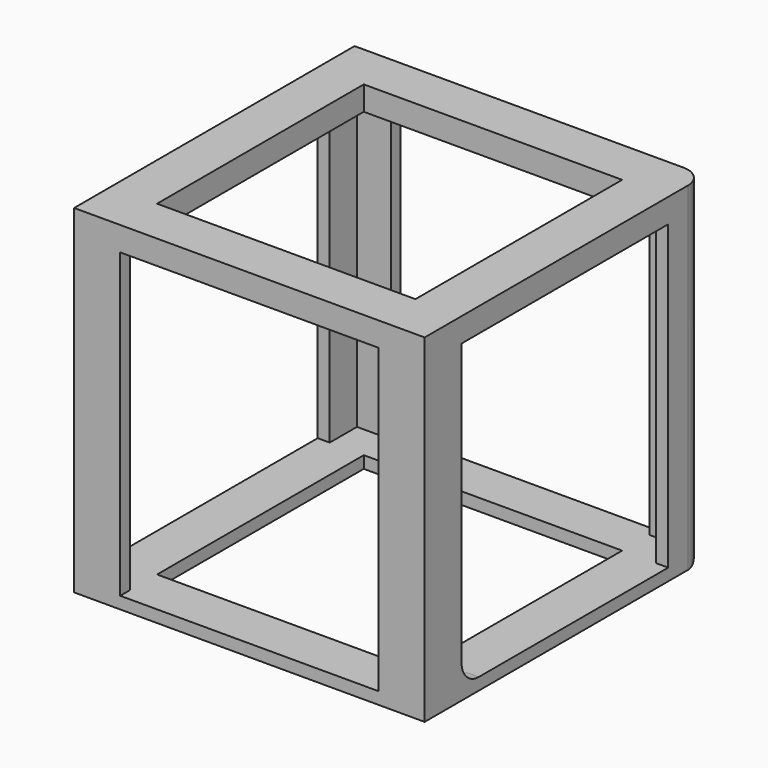
from build123d import *

# Parameters (mm, degrees)
F0_W        = 60
F0_H        = 2.8
F0_W_2      = 2.8
F0_H_2      = 60
F0_W_3      = 7.9
F0_H_3      = 7.9
F1_DEPTH    = 75.8
F2_DEPTH    = 70.2
F3_DEPTH    = 75.8
F4_DEPTH    = 2.8
F5_T1_DEPTH = 2.8
F5_T3_DEPTH = 106.4
F5_T5_DEPTH = 103.6


# Not quite as in the source:
# - a fillet or chamfer that OpenCascade refuses, or shapes differently, is made with other operations: its cross-section is extruded or revolved along the edge and cut away or added


with BuildPart() as f1:
    # F0 (on Top) → F1 (new body)
    with BuildSketch(Plane.XY):
        with Locations((0, 39.3)):
            Rectangle(F0_W, F0_H)
        Polygon((-40.7, 30), (-37.9, 30), (-37.9, 37.9), (-30, 37.9), (-30, 40.7), (-40.7, 40.7), align=None)
        Polygon((37.9, 37.9), (37.9, 30), (40.7, 30), (40.7, 40.7), (30, 40.7), (30, 37.9), align=None)
        with Locations((39.3, 0)):
            Rectangle(F0_W_2, F0_H_2)
        Polygon((37.9, -30), (37.9, -37.9), (30, -37.9), (30, -40.7), (40.7, -40.7), (40.7, -30), align=None)
        with Locations((0, -39.3)):
            Rectangle(F0_W, F0_H)
        Polygon((-30, -40.7), (-30, -37.9), (-37.9, -37.9), (-37.9, -30), (-40.7, -30), (-40.7, -40.7), align=None)
        with Locations((-39.3, 0)):
            Rectangle(F0_W_2, F0_H_2)
        with Locations((33.95, -33.95)):
            Rectangle(F0_W_3, F0_H_3)
        with Locations((33.95, 33.95)):
            Rectangle(F0_W_3, F0_H_3)
        with Locations((-33.95, 33.95)):
            Rectangle(F0_W_3, F0_H_3)
        with Locations((-33.95, 0)):
            Rectangle(F0_W_3, F0_H_2)
        with Locations((33.95, 0)):
            Rectangle(F0_W_3, F0_H_2)
        with Locations((-33.95, -33.95)):
            Rectangle(F0_W_3, F0_H_3)
        with Locations((0, -33.95)):
            Rectangle(F0_W, F0_H_3)
        with Locations((0, 33.95)):
            Rectangle(F0_W, F0_H_3)
    extrude(amount=F1_DEPTH)

    # F0 (on Top) → F2 (cut)
    with BuildSketch(Plane.XY):
        Polygon((-40.7, 30), (-37.9, 30), (-37.9, 37.9), (-30, 37.9), (-30, 40.7), (-40.7, 40.7), align=None)
        with Locations((-33.95, 33.95)):
            Rectangle(F0_W_3, F0_H_3)
        with Locations((-39.3, 0)):
            Rectangle(F0_W_2, F0_H_2)
        with Locations((-33.95, 0)):
            Rectangle(F0_W_3, F0_H_2)
        Polygon((-30, -40.7), (-30, -37.9), (-37.9, -37.9), (-37.9, -30), (-40.7, -30), (-40.7, -40.7), align=None)
        with Locations((-33.95, -33.95)):
            Rectangle(F0_W_3, F0_H_3)
        with Locations((0, -39.3)):
            Rectangle(F0_W, F0_H)
        with Locations((33.95, -33.95)):
            Rectangle(F0_W_3, F0_H_3)
        with Locations((33.95, 0)):
            Rectangle(F0_W_3, F0_H_2)
        with Locations((33.95, 33.95)):
            Rectangle(F0_W_3, F0_H_3)
        with Locations((0, 33.95)):
            Rectangle(F0_W, F0_H_3)
        with Locations((0, 39.3)):
            Rectangle(F0_W, F0_H)
        Polygon((37.9, 37.9), (37.9, 30), (40.7, 30), (40.7, 40.7), (30, 40.7), (30, 37.9), align=None)
        with Locations((39.3, 0)):
            Rectangle(F0_W_2, F0_H_2)
        Polygon((37.9, -30), (37.9, -37.9), (30, -37.9), (30, -40.7), (40.7, -40.7), (40.7, -30), align=None)
        with Locations((0, -33.95)):
            Rectangle(F0_W, F0_H_3)
    extrude(amount=F2_DEPTH, mode=Mode.SUBTRACT)

    # F0 (on Top) → F3 (join)
    with BuildSketch(Plane.XY):
        Polygon((-30, -40.7), (-30, -37.9), (-37.9, -37.9), (-37.9, -30), (-40.7, -30), (-40.7, -40.7), align=None)
        Polygon((37.9, -30), (37.9, -37.9), (30, -37.9), (30, -40.7), (40.7, -40.7), (40.7, -30), align=None)
        Polygon((37.9, 37.9), (37.9, 30), (40.7, 30), (40.7, 40.7), (30, 40.7), (30, 37.9), align=None)
        Polygon((-40.7, 30), (-37.9, 30), (-37.9, 37.9), (-30, 37.9), (-30, 40.7), (-40.7, 40.7), align=None)
    extrude(amount=F3_DEPTH)

    # F0 (on Top) → F4 (join)
    with BuildSketch(Plane.XY):
        Polygon((-30, -40.7), (-30, -37.9), (-37.9, -37.9), (-37.9, -30), (-40.7, -30), (-40.7, -40.7), align=None)
        with Locations((-33.95, -33.95)):
            Rectangle(F0_W_3, F0_H_3)
        with Locations((0, -33.95)):
            Rectangle(F0_W, F0_H_3)
        with Locations((0, -39.3)):
            Rectangle(F0_W, F0_H)
        Polygon((37.9, -30), (37.9, -37.9), (30, -37.9), (30, -40.7), (40.7, -40.7), (40.7, -30), align=None)
        with Locations((33.95, -33.95)):
            Rectangle(F0_W_3, F0_H_3)
        with Locations((39.3, 0)):
            Rectangle(F0_W_2, F0_H_2)
        with Locations((33.95, 0)):
            Rectangle(F0_W_3, F0_H_2)
        with Locations((33.95, 33.95)):
            Rectangle(F0_W_3, F0_H_3)
        Polygon((37.9, 37.9), (37.9, 30), (40.7, 30), (40.7, 40.7), (30, 40.7), (30, 37.9), align=None)
        with Locations((0, 33.95)):
            Rectangle(F0_W, F0_H_3)
        with Locations((0, 39.3)):
            Rectangle(F0_W, F0_H)
        with Locations((-33.95, 33.95)):
            Rectangle(F0_W_3, F0_H_3)
        Polygon((-40.7, 30), (-37.9, 30), (-37.9, 37.9), (-30, 37.9), (-30, 40.7), (-40.7, 40.7), align=None)
        with Locations((-39.3, 0)):
            Rectangle(F0_W_2, F0_H_2)
        with Locations((-33.95, 0)):
            Rectangle(F0_W_3, F0_H_2)
    extrude(amount=-F4_DEPTH)

    # F5: fillet of radius 5 on 3 edges, made by hand

    # F5_s2 → F5_t1 (join)
    with BuildSketch(Plane.YZ.offset(37.9)):
        with BuildLine():
            ThreePointArc((-25, 0), (-28.5355339059, 1.4644660941), (-30, 5))
            Line((-30, 5), (-30, 0))
            Line((-30, 0), (-25, 0))
        make_face()
    extrude(amount=F5_T1_DEPTH)

    # F5_s4 → F5_t3 (cut)
    with BuildSketch(Plane.YZ.offset(-53.2)):
        with BuildLine():
            ThreePointArc((40.7, 2.2), (39.2355339059, -1.3355339059), (35.7, -2.8))
            Line((35.7, -2.8), (40.7, -2.8))
            Line((40.7, -2.8), (40.7, 2.2))
        make_face()
    extrude(amount=F5_T3_DEPTH, mode=Mode.SUBTRACT)

    # F5_s6 → F5_t5 (cut)
    with BuildSketch(Plane.XY.offset(-15.3)):
        with BuildLine():
            ThreePointArc((40.7, 35.7), (39.2355339059, 39.2355339059), (35.7, 40.7))
            Line((35.7, 40.7), (40.7, 40.7))
            Line((40.7, 40.7), (40.7, 35.7))
        make_face()
    extrude(amount=F5_T5_DEPTH, mode=Mode.SUBTRACT)


solid = f1.part
